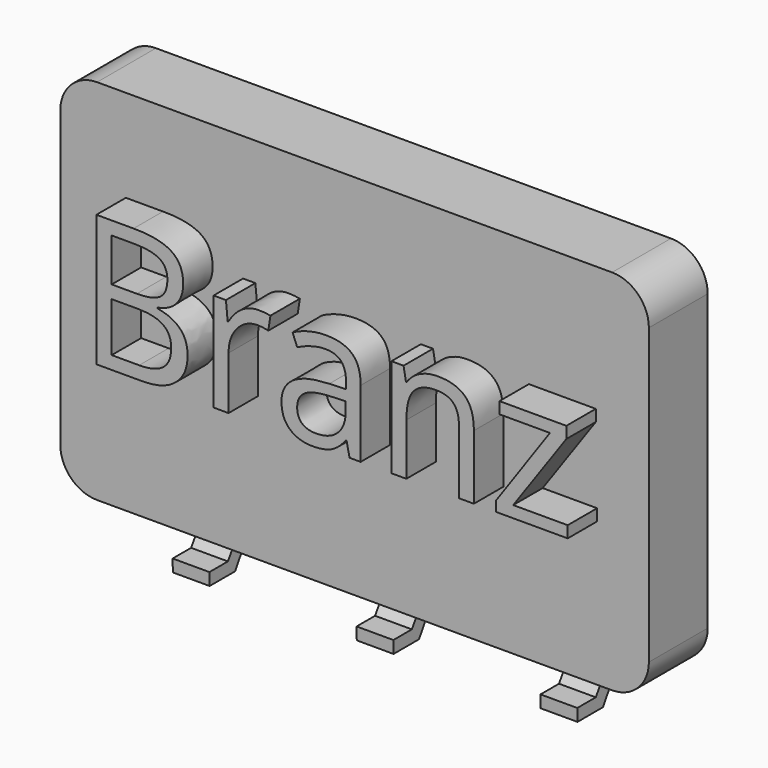
from build123d import *

# Parameters (mm, degrees)
F0_W         = 80
F0_H         = 50
F1_DEPTH     = 10
F2_TEXT_SIZE = 25.0596656568
F3_DEPTH     = 5
F4_R         = 5
F7_DEPTH     = 2.5
F11_DEPTH    = 2.5
F13_DEPTH    = 2.5


# Not quite as in the source:
# - Text() gives the source's letters only with a copy of the font that has no kerning and outlines rounded to 1/6400 em; it was checked with that copy


with BuildPart() as f1:
    # F0 (on Front) → F1 (new body)
    with BuildSketch(Plane.XZ):
        with Locations((40, 25)):
            Rectangle(F0_W, F0_H)
    extrude(amount=F1_DEPTH)

    # F2 (on face) → F3 (join)
    with BuildSketch(Plane.XZ.offset(10)):
        with Locations((6.4489371143, 19.546540454)):
            Text('Branz', F2_TEXT_SIZE, font='Open Sans', text_align=(TextAlign.LEFT, TextAlign.BOTTOM))
    extrude(amount=F3_DEPTH)

    # F4
    f4_edges = [f1.edges().sort_by_distance(p)[0] for p in [
        (0, -5, 50),
        (80, -5, 50),
        (80, -5, 0),
        (0, -5, 0),
    ]]
    fillet(f4_edges, radius=F4_R)

    # F6 (on offset) → F7 (join, symmetric)
    with BuildSketch(Plane.YZ.offset(15)):
        Polygon((0, -4.0604127571), (0, 0), (-2.1150212269, 0), (-2.1150212269, -3.986116033), (-3.3945902135, -5.96363144), (-6.5348568978, -5.96363144), (-6.5013756976, -7.6460679993), (-2.1708982531, -7.6460679993), align=None)
    extrude(amount=F7_DEPTH, both=True)

    # F9 (on offset) → F11 (join, symmetric)
    with BuildSketch(Plane.YZ.offset(40)):
        Polygon((-2.1150212269, 0), (-2.1150212269, -3.986116033), (-3.3945902135, -5.96363144), (-4.9032727141, -5.96363144), (-6.5348568978, -5.96363144), (-6.5013756976, -7.6460679993), (-2.1708982531, -7.6460679993), (0, -4.0604127571), (0, 0), align=None)
    extrude(amount=F11_DEPTH, both=True)

    # F12 (on offset) → F13 (join, symmetric)
    with BuildSketch(Plane.YZ.offset(65)):
        Polygon((-2.1150212269, 0), (-2.1150212269, -3.986116033), (-3.3945902135, -5.96363144), (-6.5348568978, -5.96363144), (-6.5013756976, -7.6460679993), (-2.1708982531, -7.6460679993), (0, -4.0604127571), (0, 0), align=None)
    extrude(amount=F13_DEPTH, both=True)


solid = f1.part
